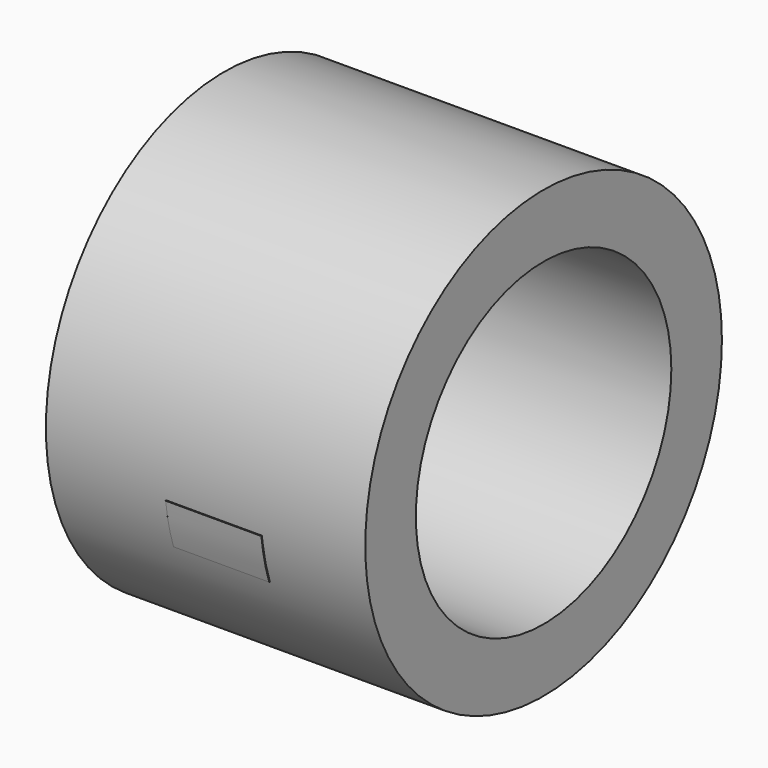
from build123d import *

# Parameters (mm, degrees)
F0_R         = 1.75
F0_R_2       = 1.745
F0_R_3       = 1.25
F1_DEPTH     = 2.5
F2_TEXT_SIZE = 2.8570699214
F3_REACH     = 2.5772511416
F4_DEPTH     = 2.5


# Not quite as in the source:
# - Text() gives the source's letters only with a copy of the font that has no kerning and outlines rounded to 1/6400 em; it was checked with that copy


with BuildPart() as f1:
    # F0 (on Right) → F1 (new body)
    with BuildSketch(Plane.YZ):
        Circle(F0_R)
        Circle(F0_R_2, mode=Mode.SUBTRACT)
        Circle(F0_R_2)
        Circle(F0_R_3, mode=Mode.SUBTRACT)
    extrude(amount=F1_DEPTH)

    f3_end = f1.faces().sort_by_distance((1.25, -1.75, 0))[0]
    # F2 (on Front) → F3 (intersect, up to a face of the model that its end follows)
    with BuildSketch(Plane.XZ):
        with Locations((0.8468861342, -1.1417980422)):
            Text('-', F2_TEXT_SIZE, font='Open Sans', font_style=FontStyle.BOLD, text_align=(TextAlign.LEFT, TextAlign.BOTTOM))
    f3_long = extrude(amount=F3_REACH, mode=Mode.PRIVATE)
    add(split(f3_long, bisect_by=f3_end, keep=Keep.BOTTOM, mode=Mode.PRIVATE), mode=Mode.INTERSECT)


with BuildPart() as f4:
    # F0 (on Right) → F4 (new body)
    with BuildSketch(Plane.YZ):
        Circle(F0_R_2)
        Circle(F0_R_3, mode=Mode.SUBTRACT)
    extrude(amount=F4_DEPTH)


solid = Compound([f1.part, f4.part])
